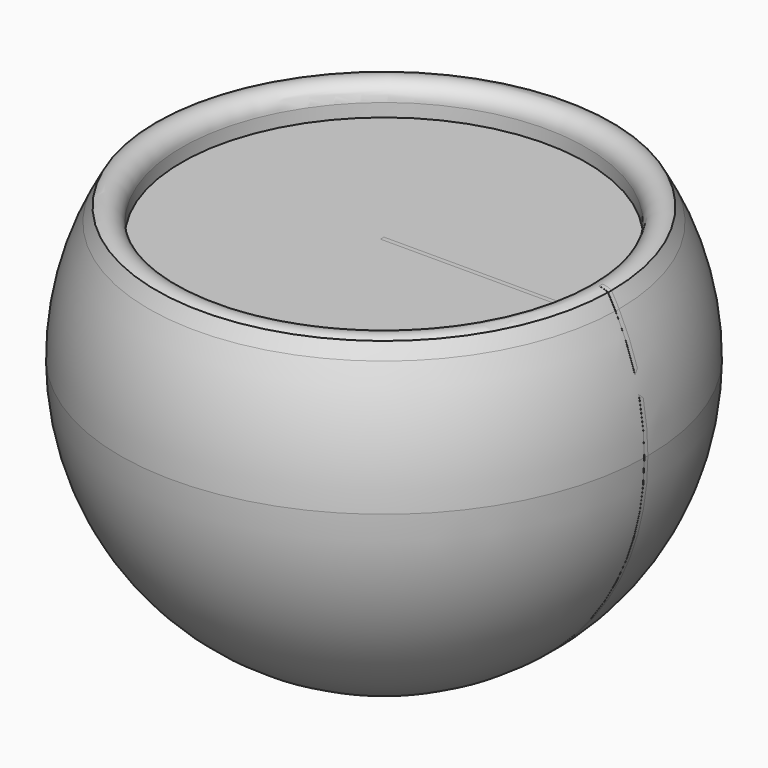
from build123d import *

# Parameters (mm, degrees)
F3_DEPTH = 1
F4_DEPTH = 1


# Not quite as in the source:
# - a feature names something its author has since deleted; it is built from what else it names


with BuildPart() as f2:
    # F0 (on Front) → F2 (revolve)
    with BuildSketch(Plane.XZ):
        with BuildLine():
            Line((0, 16.248711306), (49.3961474297, 16.248711306))
            ThreePointArc((49.3961474297, 16.248711306), (47.8655015236, 20.3197874963), (46, 24.248711306))
            Line((46, 24.248711306), (0, 24.248711306))
            Line((0, 24.248711306), (0, 16.248711306))
        make_face()
        with BuildLine():
            ThreePointArc((0, -60), (42.4264068712, -42.4264068712), (60, 0))
            Line((60, 0), (52, 0))
            ThreePointArc((52, 0), (36.7695526217, -36.7695526217), (0, -52))
            Line((0, -52), (0, -60))
        make_face()
        with BuildLine():
            Line((52, 0), (60, 0))
            ThreePointArc((60, 0), (58.3409790885, 14.0117864313), (53.4556613668, 27.248711306))
            Line((53.4556613668, 27.248711306), (46, 27.248711306))
            Line((46, 27.248711306), (46, 24.248711306))
            ThreePointArc((46, 24.248711306), (47.8655015236, 20.3197874963), (49.3961474297, 16.248711306))
            ThreePointArc((49.3961474297, 16.248711306), (51.3449104895, 8.2280111101), (52, 0))
        make_face()
        with BuildLine():
            Line((46, 27.248711306), (53.4556613668, 27.248711306))
            ThreePointArc((53.4556613668, 27.248711306), (52.6182835721, 28.8325551058), (51.7339912755, 30.3906917774))
            ThreePointArc((51.7339912755, 30.3906917774), (47.93644929, 30.5179121728), (46, 27.248711306))
        make_face()
    revolve(axis=Axis((0, 0, 0), (0, 0, 1)))


with BuildPart() as f3:
    # F0 (on Front) → F3 (new body)
    with BuildSketch(Plane.XZ):
        with BuildLine():
            Line((0, 16.248711306), (49.3961474297, 16.248711306))
            ThreePointArc((49.3961474297, 16.248711306), (47.8655015236, 20.3197874963), (46, 24.248711306))
            Line((46, 24.248711306), (0, 24.248711306))
            Line((0, 24.248711306), (0, 16.248711306))
        make_face()
        with BuildLine():
            Line((46, 27.248711306), (53.4556613668, 27.248711306))
            ThreePointArc((53.4556613668, 27.248711306), (52.6182835721, 28.8325551058), (51.7339912755, 30.3906917774))
            ThreePointArc((51.7339912755, 30.3906917774), (47.93644929, 30.5179121728), (46, 27.248711306))
        make_face()
        with BuildLine():
            Line((52, 0), (60, 0))
            ThreePointArc((60, 0), (58.3409790885, 14.0117864313), (53.4556613668, 27.248711306))
            Line((53.4556613668, 27.248711306), (46, 27.248711306))
            Line((46, 27.248711306), (46, 24.248711306))
            ThreePointArc((46, 24.248711306), (47.8655015236, 20.3197874963), (49.3961474297, 16.248711306))
            ThreePointArc((49.3961474297, 16.248711306), (51.3449104895, 8.2280111101), (52, 0))
        make_face()
    extrude(amount=F3_DEPTH)


with BuildPart() as f4:
    # F0 (on Front) → F4 (new body)
    with BuildSketch(Plane.XZ):
        with BuildLine():
            ThreePointArc((0, -60), (42.4264068712, -42.4264068712), (60, 0))
            Line((60, 0), (52, 0))
            ThreePointArc((52, 0), (36.7695526217, -36.7695526217), (0, -52))
            Line((0, -52), (0, -60))
        make_face()
    extrude(amount=F4_DEPTH)


solid = Compound([f2.part, f3.part, f4.part])
